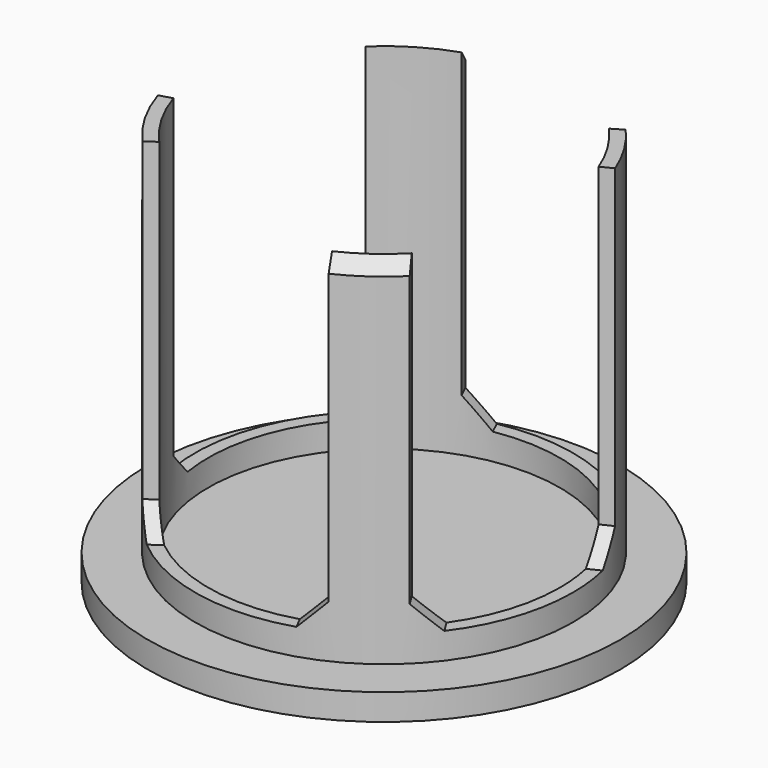
from build123d import *

# Parameters (mm, degrees)
F0_R        = 45
F1_DEPTH    = 5
F2_R        = 36
F2_R_2      = 33.5
F3_DEPTH    = 70
F5_DEPTH    = 65
F6_R        = 3.4
F7_DEPTH    = 5.001
F8_T2_ANGLE = 64.3663587264
F8_T4_ANGLE = 60.259047326
F9_SIZE     = 5


# Not quite as in the source:
# - a fillet or chamfer that OpenCascade refuses, or shapes differently, is made with other operations: its cross-section is extruded or revolved along the edge and cut away or added


with BuildPart() as f1:
    # F0 (on Top) → F1 (new body)
    with BuildSketch(Plane.XY):
        Circle(F0_R)
    extrude(amount=F1_DEPTH)

    # F2 (on face) → F3 (join)
    with BuildSketch(Plane.XY.offset(5)):
        Circle(F2_R)
        Circle(F2_R_2, mode=Mode.SUBTRACT)
    extrude(amount=F3_DEPTH)

    # F4 (on face) → F5 (cut)
    with BuildSketch(Plane.XY.offset(75)):
        with BuildLine():
            Line((-23.0004066086, 24.3563399516), (-24.2860665521, 26.5741786595))
            ThreePointArc((-24.2860665521, 26.5741786595), (-34.7900436906, 9.2548830357), (-34.2800852695, -10.9943510002))
            Line((-34.2800852695, -10.9943510002), (-31.8828522812, -10.2826908158))
            ThreePointArc((-31.8828522812, -10.2826908158), (-32.4500946026, 8.321139362), (-23.0004066086, 24.3563399516))
        make_face()
        with BuildLine():
            ThreePointArc((26.9790229265, 23.8355264664), (9.1813045472, 34.8095338494), (-11.7135995274, 34.0410279826))
            Line((-11.7135995274, 34.0410279826), (-10.6344524928, 31.7672538973))
            ThreePointArc((-10.6344524928, 31.7672538973), (8.4559678958, 32.4152218401), (24.7971983706, 22.5244079383))
            Line((24.7971983706, 22.5244079383), (26.9790229265, 23.8355264664))
        make_face()
        with BuildLine():
            ThreePointArc((36, 0), (35.3753586598, 6.6771251068), (33.5231111282, 13.1225386373))
            Line((33.5231111282, 13.1225386373), (31.2720148564, 12.012954958))
            ThreePointArc((31.2720148564, 12.012954958), (32.9382945649, 6.1089075256), (33.5, 0))
            ThreePointArc((33.5, 0), (31.0323255924, -12.619222176), (23.9928496521, -23.3793320173))
            Line((23.9928496521, -23.3793320173), (25.3486350697, -25.562603547))
            ThreePointArc((25.3486350697, -25.562603547), (33.2306399465, -13.8464641243), (36, 0))
        make_face()
        with BuildLine():
            Line((-24.739174036, -22.5881222774), (-26.8374439413, -23.9948244982))
            ThreePointArc((-26.8374439413, -23.9948244982), (-7.1064924362, -35.2916104089), (15.4589834804, -32.5118413775))
            Line((15.4589834804, -32.5118413775), (14.3252158119, -30.2826384574))
            ThreePointArc((14.3252158119, -30.2826384574), (-6.4741042843, -32.8684647301), (-24.739174036, -22.5881222774))
        make_face()
    extrude(amount=-F5_DEPTH, mode=Mode.SUBTRACT)

    # F6 (on face) → F7 (cut, through all)
    with BuildSketch(Plane.XY.offset(5)):
        Circle(F6_R)
    extrude(amount=-F7_DEPTH, mode=Mode.SUBTRACT)

    # F8: chamfer of 5 on 2 edges, made by hand

    # F8_s1 → F8_t2 (revolve, cut)
    with BuildSketch(Plane(origin=(0, 0, 0), x_dir=(0, 0, 1), z_dir=(0.9996677989, -0.0257738601, 0))):
        Polygon((70, -36), (75, -31), (75, -36), align=None)
    revolve(axis=Axis((0, 0, 75), (0, 0, 1)), revolution_arc=F8_T2_ANGLE, mode=Mode.SUBTRACT)

    # F8_s3 → F8_t4 (revolve, cut)
    with BuildSketch(Plane(origin=(0, 0, 0), x_dir=(0, 0, 1), z_dir=(-0.9962472468, -0.0865530086, 0))):
        Polygon((70, -36), (75, -31), (75, -36), align=None)
    revolve(axis=Axis((0, 0, 75), (0, 0, 1)), revolution_arc=F8_T4_ANGLE, mode=Mode.SUBTRACT)

    # F9
    f9_edges = [f1.edges().sort_by_distance(p)[0] for p in [
        (-23.643237, 25.465259, 10),
        (-11.174026, 32.904141, 10),
        (25.888111, 23.179967, 10),
        (32.397563, 12.567747, 10),
        (24.670742, -24.470968, 10),
        (14.8921, -31.39724, 10),
        (-25.788309, -23.291473, 10),
        (-33.081469, -10.638521, 10),
    ]]
    chamfer(f9_edges, length=F9_SIZE)


solid = f1.part
